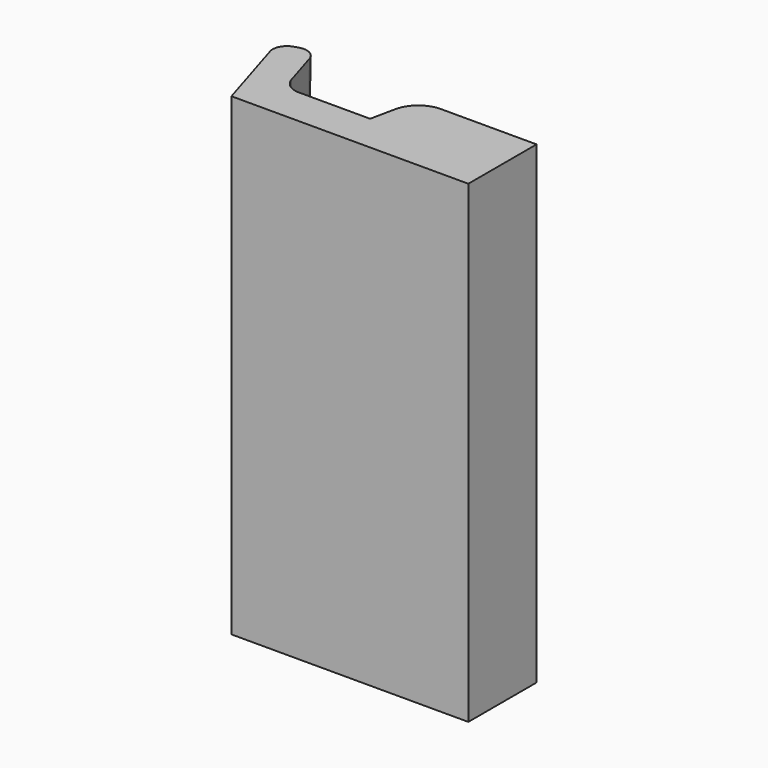
from build123d import *

# Parameters (mm, degrees)
F1_DEPTH    = 50
F2_SIZE2    = 2.49999
F2_SIZE     = 49.99999
F3_T1_DEPTH = 57.5624504994
F4_R        = 2
F5_R        = 3


# Not quite as in the source:
# - a fillet or chamfer that OpenCascade refuses, or shapes differently, is made with other operations: its cross-section is extruded or revolved along the edge and cut away or added
# - a fillet or chamfer is up to 0.001 mm smaller than in the source, because OpenCascade refuses the exact size


with BuildPart() as f1:
    # F0 (on Top) → F1 (new body)
    with BuildSketch(Plane.XY):
        Polygon((-4.0792049388, 6.6941332917), (-7.4262715846, 5.6708323252), (-4.4696014276, -4), (20.5303985724, -4), (20.5303985724, 5), (8.0088521886, 5), (6.9673969943, 0), (-2.0326030057, 0), align=None)
    extrude(amount=F1_DEPTH)

    # F2 (size 50 and 2.5 in the source; OpenCascade refuses exactly that, so slightly less here)
    f2_edges = [f1.edges().sort_by_distance(p)[0] for p in [
        (-5.752738, 6.182483, 0),
    ]]
    f2_side = f1.faces().sort_by_distance((-5.752738, 6.182483, 25))[0]
    chamfer(f2_edges, length=F2_SIZE, length2=F2_SIZE2, reference=f2_side)

    # F3: fillet of radius 1.5 on 2 edges, made by hand

    # F3_s2 → F3_t1 (cut)
    with BuildSketch(Plane(origin=(-0.7893916774, 2.5819838349, 53.9993894282), x_dir=(0.956304756, 0.2923717047, 0), z_dir=(0.0146002909, -0.0477553996, -0.9987523483))):
        with BuildLine():
            ThreePointArc((-1.9437879213, -3.5879297119), (-2.3831277496, -4.6485898837), (-3.4437879213, -5.0879297119))
            Line((-3.4437879213, -5.0879297119), (-1.9437879213, -5.0879297119))
            Line((-1.9437879213, -5.0879297119), (-1.9437879213, -3.5879297119))
        make_face()
        with BuildLine():
            ThreePointArc((-3.9437879213, -5.0879297119), (-5.0044480931, -4.6485898837), (-5.4437879213, -3.5879297119))
            Line((-5.4437879213, -3.5879297119), (-5.4437879213, -5.0879297119))
            Line((-5.4437879213, -5.0879297119), (-3.9437879213, -5.0879297119))
        make_face()
    extrude(amount=F3_T1_DEPTH, mode=Mode.SUBTRACT)

    # F4
    f4_edges = [f1.edges().sort_by_distance(p)[0] for p in [
        (-2.032603, 0, 25),
    ]]
    fillet(f4_edges, radius=F4_R)

    # F5
    f5_edges = [f1.edges().sort_by_distance(p)[0] for p in [
        (8.008852, 5, 25),
    ]]
    fillet(f5_edges, radius=F5_R)


solid = f1.part
